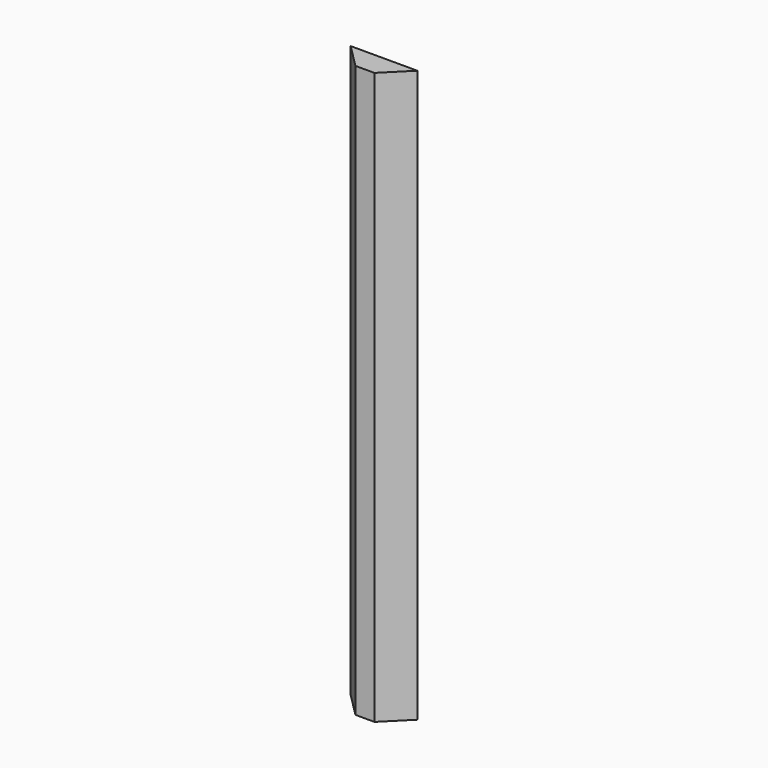
from build123d import *

# Parameters (mm, degrees)
F0_W        = 12.7
F0_H        = 76.2
F1_DEPTH    = 1.5875
F2_T1_DEPTH = 102.3282991577


# Not quite as in the source:
# - a fillet or chamfer that OpenCascade refuses, or shapes differently, is made with other operations: its cross-section is extruded or revolved along the edge and cut away or added


with BuildPart() as f1:
    # F0 (on Front) → F1 (new body, symmetric)
    with BuildSketch(Plane.XZ):
        Rectangle(F0_W, F0_H)
    extrude(amount=F1_DEPTH, both=True)

    # F2: chamfer of 5.08 on 2 edges, made by hand

    # F2_s2 → F2_t1 (cut)
    with BuildSketch(Plane.XY.offset(-51.1641495789)):
        Polygon((-6.35, 3.4925), (-1.27, -1.5875), (-6.35, -1.5875), align=None)
        Polygon((6.35, 3.4925), (1.27, -1.5875), (6.35, -1.5875), align=None)
    extrude(amount=F2_T1_DEPTH, mode=Mode.SUBTRACT)


solid = f1.part
